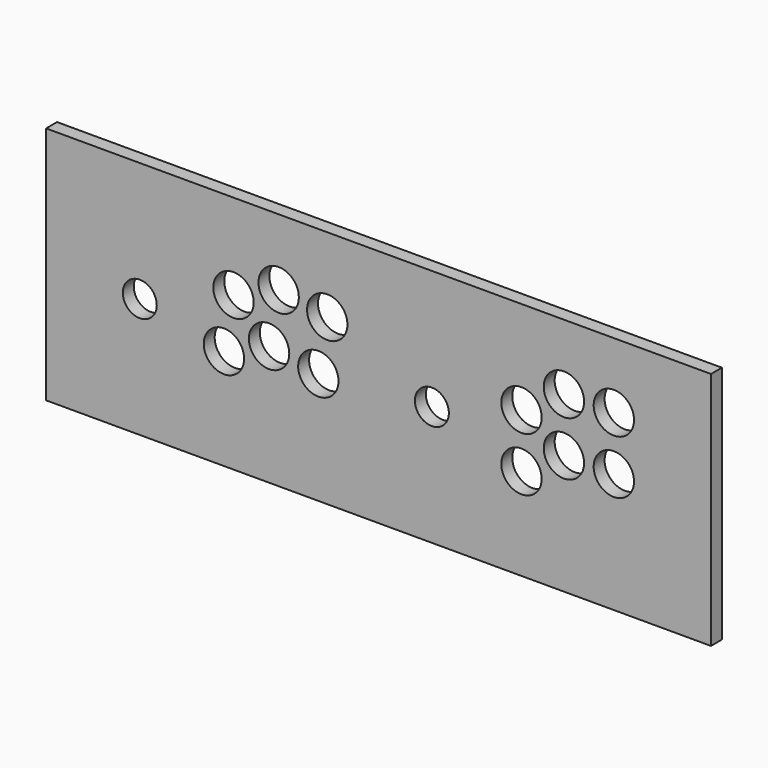
from build123d import *

# Parameters (mm, degrees)
F0_W     = 486
F0_H     = 175
F1_DEPTH = 10
F5_R     = 14.75
F5_R_2   = 12.4064380464
F7_DEPTH = 25
F3_R     = 14.75
F3_R_2   = 12.4065
F8_DEPTH = 25


# Not quite as in the source:
# - a feature names something its author has since deleted; it is built from what else it names


with BuildPart() as f1:
    # F0 (on Front) → F1 (new body)
    with BuildSketch(Plane.XZ):
        with Locations((243, 87.5)):
            Rectangle(F0_W, F0_H)
    extrude(amount=F1_DEPTH)

    # F5 (on face) → F7 (cut)
    with BuildSketch(Plane.XZ.offset(10)):
        with Locations((347.5, 106.75)):
            Circle(F5_R)
        with Locations((378.5, 127)):
            Circle(F5_R)
        with Locations((415, 127)):
            Circle(F5_R)
        with Locations((415, 87.5)):
            Circle(F5_R)
        with Locations((378.5, 87.5)):
            Circle(F5_R)
        with Locations((347.5, 67.25)):
            Circle(F5_R)
        with Locations((282, 87.5)):
            Circle(F5_R_2)
    extrude(amount=-F7_DEPTH, mode=Mode.SUBTRACT)

    # F3 (on face) → F8 (cut)
    with BuildSketch(Plane.XZ.offset(10)):
        with Locations((170, 126.3350188136)):
            Circle(F3_R)
        with Locations((205.5, 120.3350188136)):
            Circle(F3_R)
        with Locations((199, 81.8350188136)):
            Circle(F3_R)
        with Locations((163, 87.8350188136)):
            Circle(F3_R)
        with Locations((130, 73.8350188136)):
            Circle(F3_R)
        with Locations((137, 112.3350188136)):
            Circle(F3_R)
        with Locations((68.5, 87.5)):
            Circle(F3_R_2)
    extrude(amount=-F8_DEPTH, mode=Mode.SUBTRACT)


solid = f1.part
